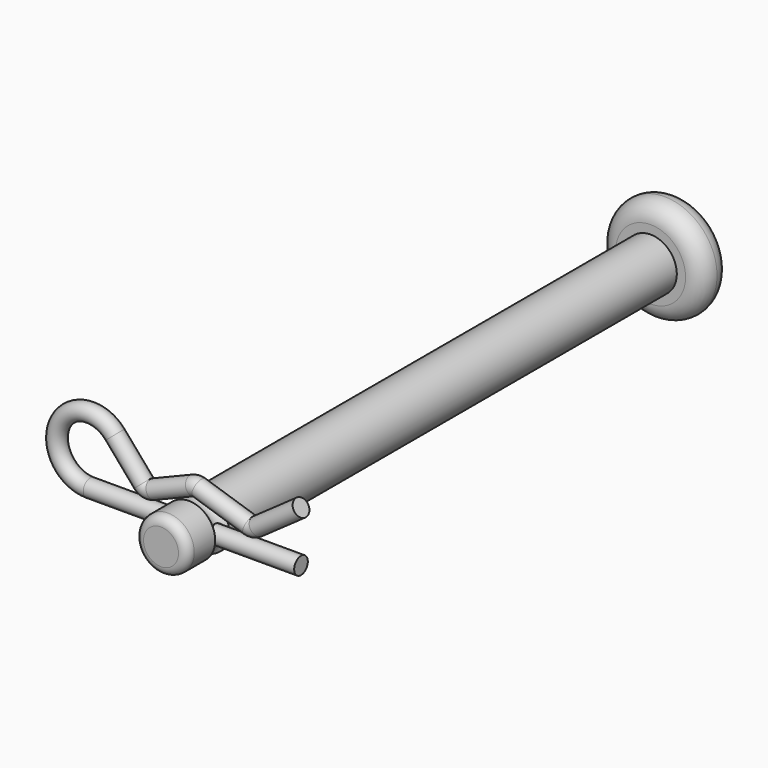
from build123d import *

# Parameters (mm, degrees)
F0_R     = 3
F1_DEPTH = 70
F0_R_2   = 6
F2_DEPTH = 4
F3_R     = 1.99999
F4_R     = 1
F5_R     = 1
F6_DEPTH = 3
F11_R    = 0.975


# Not quite as in the source:
# - a fillet or chamfer is up to 0.001 mm smaller than in the source, because OpenCascade refuses the exact size


with BuildPart() as f1:
    # F0 (on Front) → F1 (new body)
    with BuildSketch(Plane.XZ):
        Circle(F0_R)
    extrude(amount=F1_DEPTH)

    # F0 (on Front) → F2 (join)
    with BuildSketch(Plane.XZ):
        Circle(F0_R_2)
        Circle(F0_R, mode=Mode.SUBTRACT)
        Circle(F0_R)
    extrude(amount=-F2_DEPTH)

    # F3 (radius 2 in the source; OpenCascade refuses exactly that, so slightly less here)
    f3_edges = [f1.edges().sort_by_distance(p)[0] for p in [
        (-6, 4, 0),
        (-6, 0, 0),
    ]]
    fillet(f3_edges, radius=F3_R)

    # F4
    f4_edges = [f1.edges().sort_by_distance(p)[0] for p in [
        (-3, -70, 0),
    ]]
    fillet(f4_edges, radius=F4_R)

    # F5 (on Right) → F6 (cut, symmetric)
    with BuildSketch(Plane.YZ):
        with Locations((-65, 0)):
            Circle(F5_R)
    extrude(amount=F6_DEPTH, both=True, mode=Mode.SUBTRACT)

    # F5 (on Right) → F7 (revolve, cut)
    with BuildSketch(Plane.YZ):
        with BuildLine():
            ThreePointArc((-66, 3), (-65, 2.3819660113), (-64, 3))
            Line((-64, 3), (-66, 3))
        make_face()
    revolve(axis=Axis((0, -46.4799346625, 0), (0, -1, 0)), mode=Mode.SUBTRACT)


with BuildPart() as f12:
    # F12: sweep along a path in F9
    with BuildLine(Plane.XZ.offset(65)) as f12_path:
        Line((12.010208331, 0), (-12.1146072416, 0))
        ThreePointArc((-12.1146072416, 0), (-15.5566823668, 5.3660576736), (-9.2441216111, 6.2571428716))
        Line((-9.2441216111, 6.2571428716), (-5.987928152, 2.4732185361))
        ThreePointArc((-5.987928152, 2.4732185361), (-5.4636368252, 2.1531800014), (-4.8511713594, 2.2))
        Line((-4.8511713594, 2.2), (-0.3378994762, 4.0471280022))
        ThreePointArc((-0.3378994762, 4.0471280022), (0.002478886, 4.1209005021), (0.347514332, 4.0734626238))
        Line((0.347514332, 4.0734626238), (6.1627862583, 2.2))
        ThreePointArc((6.1627862583, 2.2), (6.6199541782, 2.1632187268), (7.0454582218, 2.3343960558))
        Line((7.0454582218, 2.3343960558), (12.010208331, 5.8329802886))
    # F11 (on line) → F12 (sweep)
    with BuildSketch(Plane(origin=(12.010208331, 0, 0), x_dir=(0, -1, 0), z_dir=(-1, 0, 0))):
        with Locations((65, 0)):
            Circle(F11_R)
    sweep(path=f12_path.line)


solid = Compound([f1.part, f12.part])
